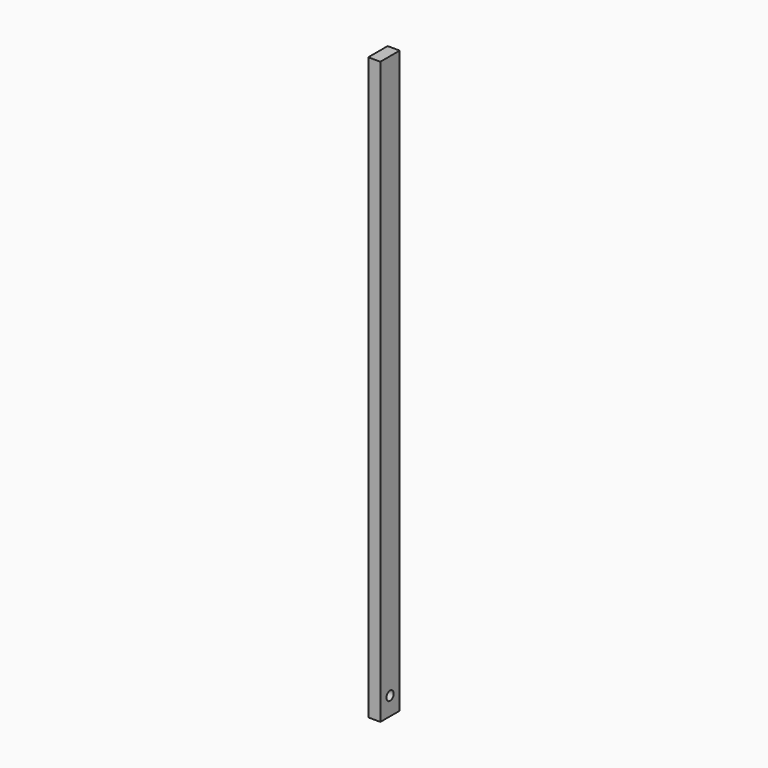
from build123d import *

# Parameters (mm, degrees)
F0_W     = 25.4
F0_H     = 50.8
F1_DEPTH = 1219.2
F3_D     = 19.05


# Not quite as in the source:
# - a feature names something its author has since deleted; it is built from what else it names


with BuildPart() as f1:
    # F0 (on Top) → F1 (new body)
    with BuildSketch(Plane.XY):
        with Locations((0.3949962629, 0)):
            Rectangle(F0_W, F0_H)
    extrude(amount=F1_DEPTH)

    # F3 (through all)
    with Locations(Plane.YZ.offset(13.0949962629)):
        with Locations((0, 38.1)):
            Hole(F3_D / 2)


solid = f1.part
